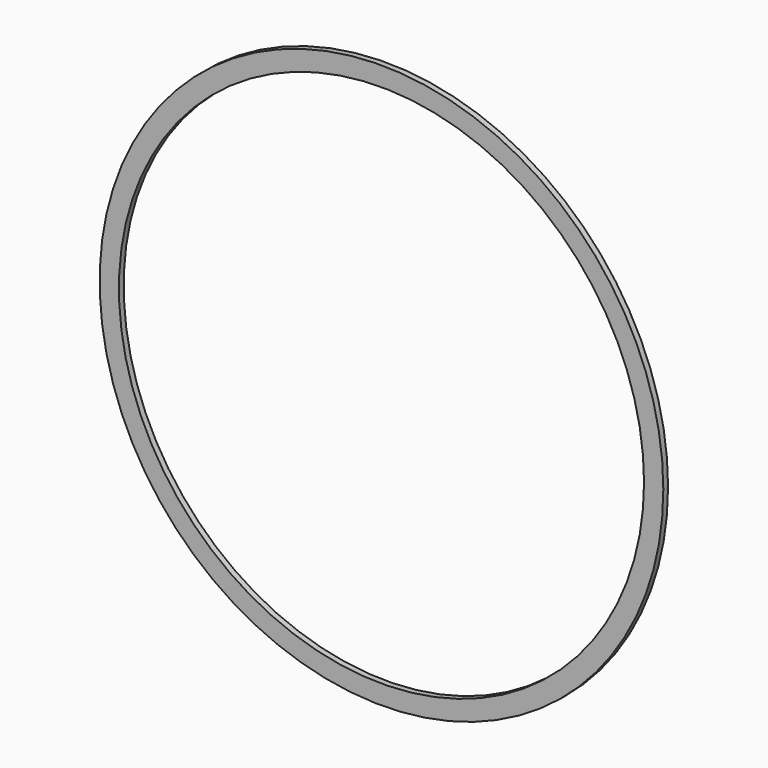
from build123d import *

# Parameters (mm, degrees)
F0_R     = 95
F0_R_2   = 88.5
F1_DEPTH = 2


# Not quite as in the source:
# - the program builds the solid bodies; features that only make, move or delete a surface that nothing else refers to are left out


with BuildPart() as f1:
    # F0 (on Front) → F1 (new body)
    with BuildSketch(Plane.XZ):
        Circle(F0_R)
        Circle(F0_R_2, mode=Mode.SUBTRACT)
    extrude(amount=F1_DEPTH)


solid = f1.part
